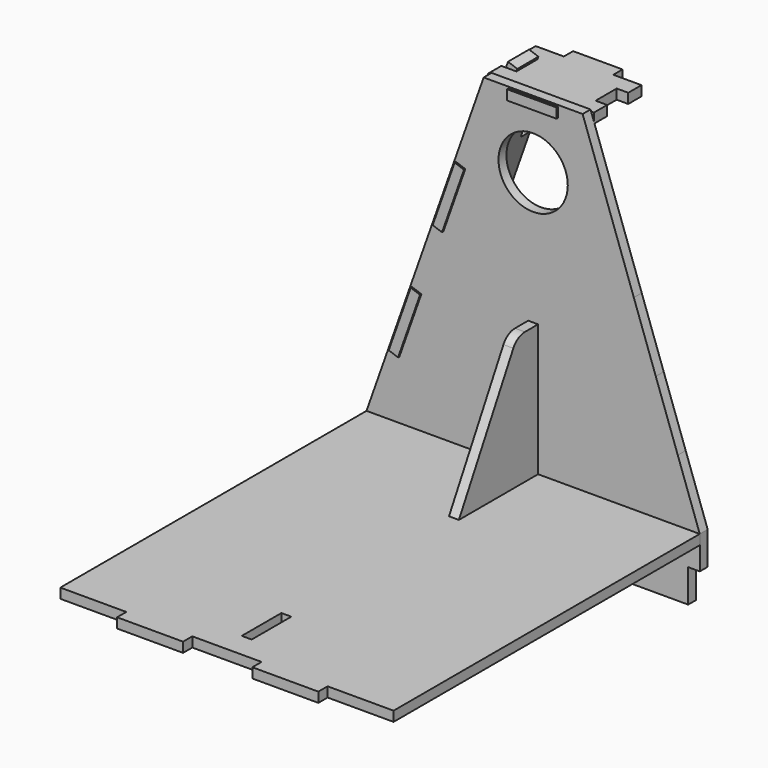
from build123d import *

# Parameters (mm, degrees)
F0_W      = 20
F0_H      = 3
F0_W_2    = 3
F0_H_2    = 10
F0_R      = 10.5
F1_DEPTH  = 3
F0_W_3    = 15
F0_H_3    = 3.5
F2_DEPTH  = 3
F4_DEPTH  = 3
F6_DEPTH  = 3
F8_DEPTH  = 3
F9_W      = 3
F9_H      = 15
F10_DEPTH = 3


# Not quite as in the source:
# - a pattern or mirror of a feature is missing from the dataset's text; its kind, count and spacing are read off the source's solid


with BuildPart() as f1:
    # F0 (on Front) → F1 (new body)
    with BuildSketch(Plane.XZ):
        with BuildLine():
            Line((23.8547611875, -4.5677042069), (15, 20.5))
            Line((15, 20.5), (7.5, 20.5))
            Line((7.5, 20.5), (7.5, 17))
            Line((7.5, 17), (-7.5, 17))
            Line((-7.5, 17), (-7.5, 20.5))
            Line((-7.5, 20.5), (-15, 20.5))
            Line((-15, 20.5), (-23.8547611875, -4.5677042069))
            Line((-23.8547611875, -4.5677042069), (-20.5545982465, -5.7334334049))
            Line((-20.5545982465, -5.7334334049), (-27.2159079497, -24.5915073532))
            Line((-27.2159079497, -24.5915073532), (-30.5160708906, -23.4257781551))
            Line((-30.5160708906, -23.4257781551), (-37.1773805937, -42.2838521034))
            Line((-37.1773805937, -42.2838521034), (-33.8772176528, -43.4495813015))
            Line((-33.8772176528, -43.4495813015), (-40.5385273559, -62.3076552498))
            Line((-40.5385273559, -62.3076552498), (-43.8386902969, -61.1419260517))
            Line((-43.8386902969, -61.1419260517), (-50.5, -80))
            Line((-50.5, -80), (-50.5, -90))
            Line((-50.5, -90), (-47, -90))
            Line((-47, -90), (-47, -100))
            Line((-47, -100), (-5, -100))
            Line((-5, -100), (-5, -95))
            ThreePointArc((-5, -95), (0, -90), (5, -95))
            Line((5, -95), (5, -100))
            Line((5, -100), (47, -100))
            Line((47, -100), (47, -90))
            Line((47, -90), (50.5, -90))
            Line((50.5, -90), (50.5, -80))
            Line((50.5, -80), (43.8386902969, -61.1419260517))
            Line((43.8386902969, -61.1419260517), (40.5385273559, -62.3076552498))
            Line((40.5385273559, -62.3076552498), (33.8772176528, -43.4495813015))
            Line((33.8772176528, -43.4495813015), (37.1773805937, -42.2838521034))
            Line((37.1773805937, -42.2838521034), (30.5160708906, -23.4257781551))
            Line((30.5160708906, -23.4257781551), (27.2159079497, -24.5915073532))
            Line((27.2159079497, -24.5915073532), (20.5545982465, -5.7334334049))
            Line((20.5545982465, -5.7334334049), (23.8547611875, -4.5677042069))
        make_face()
        with Locations((-20.5, -81.5)):
            Rectangle(F0_W, F0_H, mode=Mode.SUBTRACT)
        with Locations((20.5, -81.5)):
            Rectangle(F0_W, F0_H, mode=Mode.SUBTRACT)
        with Locations((0, -65)):
            Rectangle(F0_W_2, F0_H_2, mode=Mode.SUBTRACT)
        with Locations((0, -45)):
            Rectangle(F0_W_2, F0_H_2, mode=Mode.SUBTRACT)
        Circle(F0_R, mode=Mode.SUBTRACT)
    extrude(amount=F1_DEPTH)


with BuildPart() as f2:
    # F0 (on Front) → F2 (new body)
    with BuildSketch(Plane.XZ):
        with BuildLine():
            Line((23.8547611875, -4.5677042069), (15, 20.5))
            Line((15, 20.5), (7.5, 20.5))
            Line((7.5, 20.5), (7.5, 17))
            Line((7.5, 17), (-7.5, 17))
            Line((-7.5, 17), (-7.5, 20.5))
            Line((-7.5, 20.5), (-15, 20.5))
            Line((-15, 20.5), (-23.8547611875, -4.5677042069))
            Line((-23.8547611875, -4.5677042069), (-20.5545982465, -5.7334334049))
            Line((-20.5545982465, -5.7334334049), (-27.2159079497, -24.5915073532))
            Line((-27.2159079497, -24.5915073532), (-30.5160708906, -23.4257781551))
            Line((-30.5160708906, -23.4257781551), (-37.1773805937, -42.2838521034))
            Line((-37.1773805937, -42.2838521034), (-33.8772176528, -43.4495813015))
            Line((-33.8772176528, -43.4495813015), (-40.5385273559, -62.3076552498))
            Line((-40.5385273559, -62.3076552498), (-43.8386902969, -61.1419260517))
            Line((-43.8386902969, -61.1419260517), (-50.5, -80))
            Line((-50.5, -80), (-50.5, -90))
            Line((-50.5, -90), (-47, -90))
            Line((-47, -90), (-47, -100))
            Line((-47, -100), (-5, -100))
            Line((-5, -100), (-5, -95))
            ThreePointArc((-5, -95), (0, -90), (5, -95))
            Line((5, -95), (5, -100))
            Line((5, -100), (47, -100))
            Line((47, -100), (47, -90))
            Line((47, -90), (50.5, -90))
            Line((50.5, -90), (50.5, -80))
            Line((50.5, -80), (43.8386902969, -61.1419260517))
            Line((43.8386902969, -61.1419260517), (40.5385273559, -62.3076552498))
            Line((40.5385273559, -62.3076552498), (33.8772176528, -43.4495813015))
            Line((33.8772176528, -43.4495813015), (37.1773805937, -42.2838521034))
            Line((37.1773805937, -42.2838521034), (30.5160708906, -23.4257781551))
            Line((30.5160708906, -23.4257781551), (27.2159079497, -24.5915073532))
            Line((27.2159079497, -24.5915073532), (20.5545982465, -5.7334334049))
            Line((20.5545982465, -5.7334334049), (23.8547611875, -4.5677042069))
        make_face()
        with Locations((-20.5, -81.5)):
            Rectangle(F0_W, F0_H, mode=Mode.SUBTRACT)
        with Locations((20.5, -81.5)):
            Rectangle(F0_W, F0_H, mode=Mode.SUBTRACT)
        with Locations((0, -65)):
            Rectangle(F0_W_2, F0_H_2, mode=Mode.SUBTRACT)
        with Locations((0, -45)):
            Rectangle(F0_W_2, F0_H_2, mode=Mode.SUBTRACT)
        Circle(F0_R, mode=Mode.SUBTRACT)
        Polygon((30.5160708906, -23.4257781551), (23.8547611875, -4.5677042069), (20.5545982465, -5.7334334049), (27.2159079497, -24.5915073532), align=None)
        with Locations((0, 18.75)):
            Rectangle(F0_W_3, F0_H_3)
        Polygon((43.8386902969, -61.1419260517), (37.1773805937, -42.2838521034), (33.8772176528, -43.4495813015), (40.5385273559, -62.3076552498), align=None)
        Polygon((-20.5545982465, -5.7334334049), (-23.8547611875, -4.5677042069), (-30.5160708906, -23.4257781551), (-27.2159079497, -24.5915073532), align=None)
        Polygon((-33.8772176528, -43.4495813015), (-37.1773805937, -42.2838521034), (-43.8386902969, -61.1419260517), (-40.5385273559, -62.3076552498), align=None)
        with BuildLine():
            Line((-5, -100), (5, -100))
            Line((5, -100), (5, -95))
            ThreePointArc((5, -95), (0, -90), (-5, -95))
            Line((-5, -95), (-5, -100))
        make_face()
    extrude(amount=F2_DEPTH)


with BuildPart() as f4:
    # F3 (on face) → F4 (new body)
    with BuildSketch(Plane(origin=(-16.4738456854, 0, 5.8191196202), x_dir=(0, -1, 0), z_dir=(-0.9429036974, 0, 0.3330654852))):
        Polygon((0, 11.8579239963), (-5, 11.8579239963), (-5, 15.8579239963), (-9, 15.8579239963), (-9, -95.0157843856), (-5, -95.0157843856), (-5, -91.0157843856), (0, -91.0157843856), (0, -72.2521027935), (3.5, -72.2521027935), (3.5, -52.2521027935), (0, -52.2521027935), (0, -32.2521027935), (3.5, -32.2521027935), (3.5, -12.2521027935), (0, -12.2521027935), align=None)
    extrude(amount=F4_DEPTH)

    # F4_copies: F4 across plane


with BuildPart() as f4_1:
    add(f4.part)
    add(f4.part.mirror(Plane.ZX.offset(9)))


with BuildPart() as f6:
    # F5 (on face) → F6 (new body)
    with BuildSketch(Plane.XY.offset(17)):
        Polygon((-16.0243804767, 0), (-7.5, 0), (-7.5, -3.5), (7.5, -3.5), (7.5, 0), (16.0243804767, 0), (16.0243804767, 5), (12.5243804767, 5), (12.5243804767, 13), (16.0243804767, 13), (16.0243804767, 18), (7.5, 18), (7.5, 21.5), (-7.5, 21.5), (-7.5, 18), (-16.0243804767, 18), (-16.0243804767, 13), (-12.5243804767, 13), (-12.5243804767, 5), (-16.0243804767, 5), align=None)
    extrude(amount=F6_DEPTH)


with BuildPart() as f8:
    # F7 (on face) → F8 (new body)
    with BuildSketch(Plane(origin=(1.5, 0, 0), x_dir=(0, -1, 0), z_dir=(-1, 0, 0))):
        with BuildLine():
            ThreePointArc((12.3789206904, -42.5864852212), (10.5428749582, -40.6949115053), (8, -40))
            Line((8, -40), (-0.5, -40))
            Line((-0.5, -40), (-0.5, -50))
            Line((-0.5, -50), (3, -50))
            Line((3, -50), (3, -60))
            Line((3, -60), (-0.5, -60))
            Line((-0.5, -60), (-0.5, -70))
            Line((-0.5, -70), (3, -70))
            Line((3, -70), (3, -80))
            Line((3, -80), (10.5, -80))
            Line((10.5, -80), (10.5, -83.5))
            Line((10.5, -83.5), (25.5, -83.5))
            Line((25.5, -83.5), (25.5, -80))
            Line((25.5, -80), (33, -80))
            Line((33, -80), (12.3789206904, -42.5864852212))
        make_face()
    extrude(amount=F8_DEPTH)


with BuildPart() as f10:
    # F9 (on face) → F10 (new body)
    with BuildSketch(Plane.XY.offset(-83)):
        Polygon((-30.5, -3), (-50.5, -3), (-50.5, -119), (-30.5, -119), (-30.5, -122.5), (-10.5, -122.5), (-10.5, -119), (10.5, -119), (10.5, -122.5), (30.5, -122.5), (30.5, -119), (50.5, -119), (50.5, -3), (30.5, -3), (30.5, 0.5), (10.5, 0.5), (10.5, -3), (-10.5, -3), (-10.5, 0.5), (-30.5, 0.5), align=None)
        with Locations((0, -104)):
            Rectangle(F9_W, F9_H, mode=Mode.SUBTRACT)
        with Locations((0, -18)):
            Rectangle(F9_W, F9_H, mode=Mode.SUBTRACT)
    extrude(amount=F10_DEPTH)


solid = Compound([f1.part, f2.part, f4_1.part, f6.part, f8.part, f10.part])
